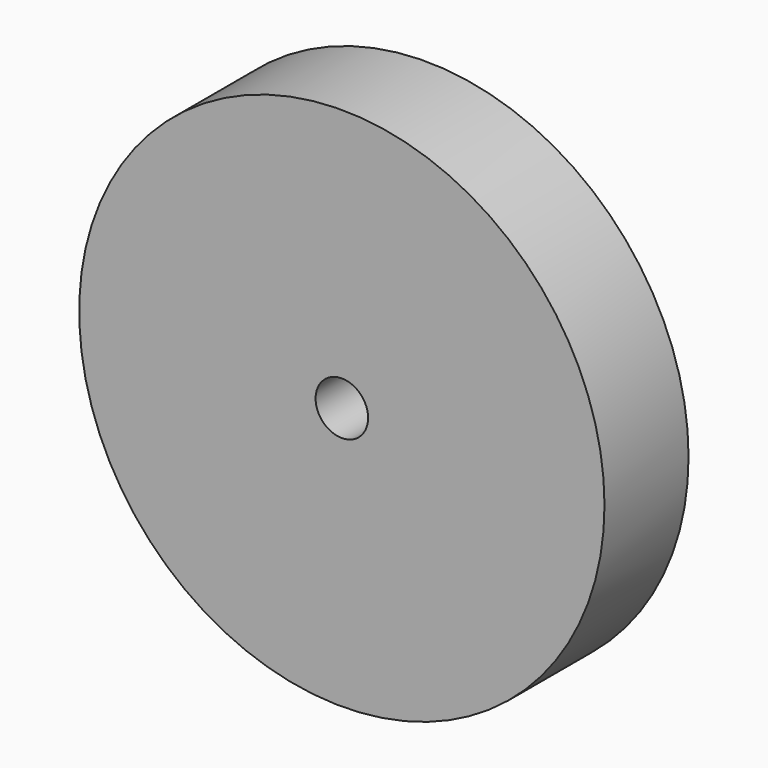
from build123d import *

# Parameters (mm, degrees)
F2_W = 22.5
F2_H = 10


# Not quite as in the source:
# - a feature of the source that left no trace in its solid (it failed there, or was rolled back) is left out


with BuildPart() as f3:
    # F2 (on Top) → F3 (revolve)
    with BuildSketch(Plane.XY):
        with Locations((13.75, 0)):
            Rectangle(F2_W, F2_H)
    revolve(axis=Axis((0, 0.6839819398, 0), (0, -1, 0)))


solid = f3.part
